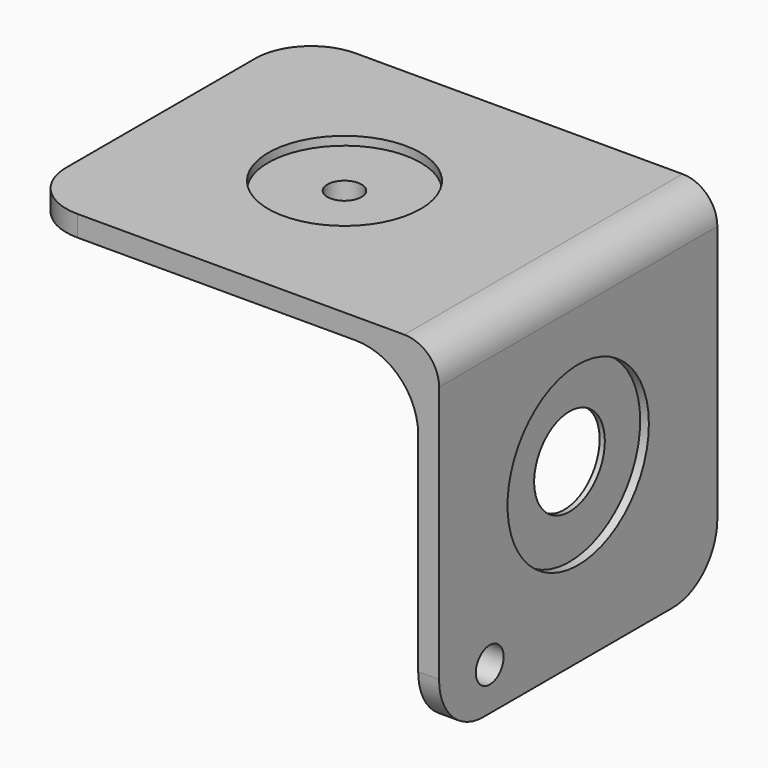
from build123d import *

# Parameters (mm, degrees)
F1_DEPTH  = 25
F2_R      = 8
F3_R      = 10.95
F3_R_2    = 2.45
F5_DEPTH  = 1.25
F6_DEPTH  = 3
F4_R      = 12.7
F4_R_2    = 6.35
F8_DEPTH  = 1.25
F7_R      = 6.35
F9_DEPTH  = 1
F10_DEPTH = 3
F11_R     = 5
F7_R_2    = 2.5
F12_DEPTH = 3
F7_R_3    = 4.5
F13_DEPTH = 1
F14_R     = 0.99999
F15_R     = 12.5
F15_R_2   = 2.45
F16_DEPTH = 1
F17_R     = 0.99999


# Not quite as in the source:
# - a fillet or chamfer is up to 0.001 mm smaller than in the source, because OpenCascade refuses the exact size


with BuildPart() as f1:
    # F0 (on Front) → F1 (new body, symmetric)
    with BuildSketch(Plane.XZ):
        with BuildLine():
            Line((30, -25), (30, 25))
            Line((30, 25), (-30, 25))
            Line((-30, 25), (-30, 22))
            Line((-30, 22), (18, 22))
            ThreePointArc((18, 22), (24.3639610307, 19.3639610307), (27, 13))
            Line((27, 13), (27, -25))
            Line((27, -25), (30, -25))
        make_face()
    extrude(amount=F1_DEPTH, both=True)

    # F2
    f2_edges = [f1.edges().sort_by_distance(p)[0] for p in [
        (-30, -25, 23.5),
        (-30, 25, 23.5),
        (28.5, 25, -25),
        (28.5, -25, -25),
    ]]
    fillet(f2_edges, radius=F2_R)

    # F3 (on face) → F5 (cut)
    with BuildSketch(Plane.XY.offset(25)):
        with Locations((-3.6, 0)):
            Circle(F3_R)
        with Locations((-3.6, 0)):
            Circle(F3_R_2, mode=Mode.SUBTRACT)
    extrude(amount=-F5_DEPTH, mode=Mode.SUBTRACT)

    # F6 (cut): a face of the model
    f6_faces = [f1.faces().sort_by_distance(p)[0] for p in [
        (-3.6, 0, 25),
    ]]
    extrude(f6_faces, amount=-F6_DEPTH, mode=Mode.SUBTRACT)

    # F4 (on face) → F8 (cut)
    with BuildSketch(Plane.YZ.offset(30)):
        Circle(F4_R)
        Circle(F4_R_2, mode=Mode.SUBTRACT)
    extrude(amount=-F8_DEPTH, mode=Mode.SUBTRACT)

    # F7 (on face) → F9 (cut)
    with BuildSketch(Plane(origin=(27, 0, 0), x_dir=(0, -1, 0), z_dir=(-1, 0, 0))):
        with BuildLine():
            ThreePointArc((0, -12.7), (8.9802561211, -8.9802561211), (12.7, 0))
            ThreePointArc((12.7, 0), (-8.9802561211, 8.9802561211), (0, -12.7))
        make_face()
        Circle(F7_R, mode=Mode.SUBTRACT)
    extrude(amount=-F9_DEPTH, mode=Mode.SUBTRACT)

    # F10 (cut): a face of the model
    f10_faces = [f1.faces().sort_by_distance(p)[0] for p in [
        (30, 0, 0),
    ]]
    extrude(f10_faces, amount=-F10_DEPTH, mode=Mode.SUBTRACT)

    # F11
    f11_edges = [f1.edges().sort_by_distance(p)[0] for p in [
        (30, 0, 25),
    ]]
    fillet(f11_edges, radius=F11_R)

    # F7 (on face) → F12 (cut)
    with BuildSketch(Plane(origin=(27, 0, 0), x_dir=(0, -1, 0), z_dir=(-1, 0, 0))):
        with Locations((15.8969778568, -18.85)):
            Circle(F7_R_2)
    extrude(amount=-F12_DEPTH, mode=Mode.SUBTRACT)

    # F7 (on face) → F13 (join)
    with BuildSketch(Plane(origin=(27, 0, 0), x_dir=(0, -1, 0), z_dir=(-1, 0, 0))):
        with Locations((15.8969778568, -18.85)):
            Circle(F7_R_3)
        with Locations((15.8969778568, -18.85)):
            Circle(F7_R_2, mode=Mode.SUBTRACT)
    extrude(amount=F13_DEPTH)

    # F14 (radius 1 in the source; OpenCascade refuses exactly that, so slightly less here)
    f14_edges = [f1.edges().sort_by_distance(p)[0] for p in [
        (26, -11.396978, -18.85),
    ]]
    fillet(f14_edges, radius=F14_R)

    # F15 (on face) → F16 (join)
    with BuildSketch(Plane(origin=(0, 0, 22), x_dir=(1, 0, 0), z_dir=(0, 0, -1))):
        with Locations((-3.6, 0)):
            Circle(F15_R)
        with Locations((-3.6, 0)):
            Circle(F15_R_2, mode=Mode.SUBTRACT)
    extrude(amount=F16_DEPTH)

    # F17 (radius 1 in the source; OpenCascade refuses exactly that, so slightly less here)
    f17_edges = [f1.edges().sort_by_distance(p)[0] for p in [
        (-16.1, 0, 21),
    ]]
    fillet(f17_edges, radius=F17_R)


solid = f1.part
